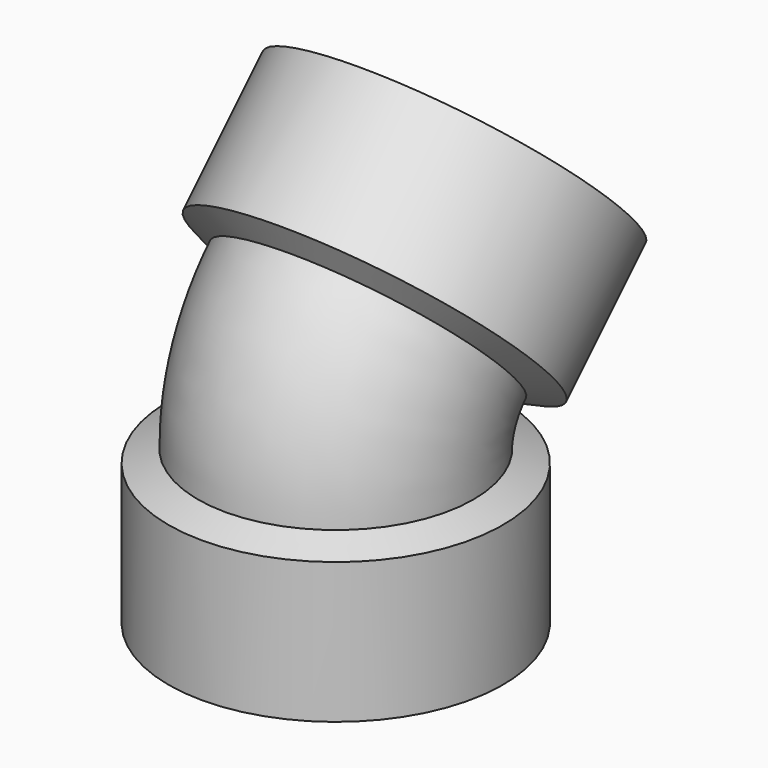
from build123d import *

# Parameters (mm, degrees)
F1_R   = 76.2
F1_R_2 = 69.088
F7_R   = 7.62
F8_R   = 7.62


with BuildPart() as f4:
    # F0 (on Right) → F4 (revolve)
    with BuildSketch(Plane.YZ):
        Polygon((-76.2, 0), (-92.47505, -7.112), (-92.47505, -84.8995), (-85.36305, -84.8995), (-85.36305, -11.7655417155), (-76.2, -7.7613996945), align=None)
    revolve(axis=Axis((0, 0, -46.00575), (0, 0, -1)))

    # F8
    f8_edges = [f4.edges().sort_by_distance(p)[0] for p in [
        (0, 76.2, -7.7614),
    ]]
    fillet(f8_edges, radius=F8_R)


with BuildPart() as f5:
    # F5: sweep along a path in F2
    with BuildLine(Plane.YZ) as f5_path:
        ThreePointArc((22.3184632736, 53.8815367264), (5.8003796226, 29.1604775462), (0, 0))
    # F1 (on Top) → F5 (sweep)
    with BuildSketch(Plane.XY):
        Circle(F1_R)
        Circle(F1_R_2, mode=Mode.SUBTRACT)
    sweep(path=f5_path.line)


with BuildPart() as f6:
    # F3 (on Right) → F6 (revolve)
    with BuildSketch(Plane.YZ):
        Polygon((16.5261881161, 178.8687314601), (-38.4778806255, 123.8646627185), (-31.5630734528, 107.7630734528), (-26.2731860569, 113.0529608487), (-30.1663061311, 122.1183503573), (21.7304941317, 174.0151506201), align=None)
    revolve(axis=Axis((0, 54.8494410722, 86.412514525), (0, 0.7071067812, 0.7071067812)))

    # F7
    f7_edges = [f6.edges().sort_by_distance(p)[0] for p in [
        (0, 81.489887, 5.289887),
    ]]
    fillet(f7_edges, radius=F7_R)


solid = Compound([f4.part, f5.part, f6.part])
